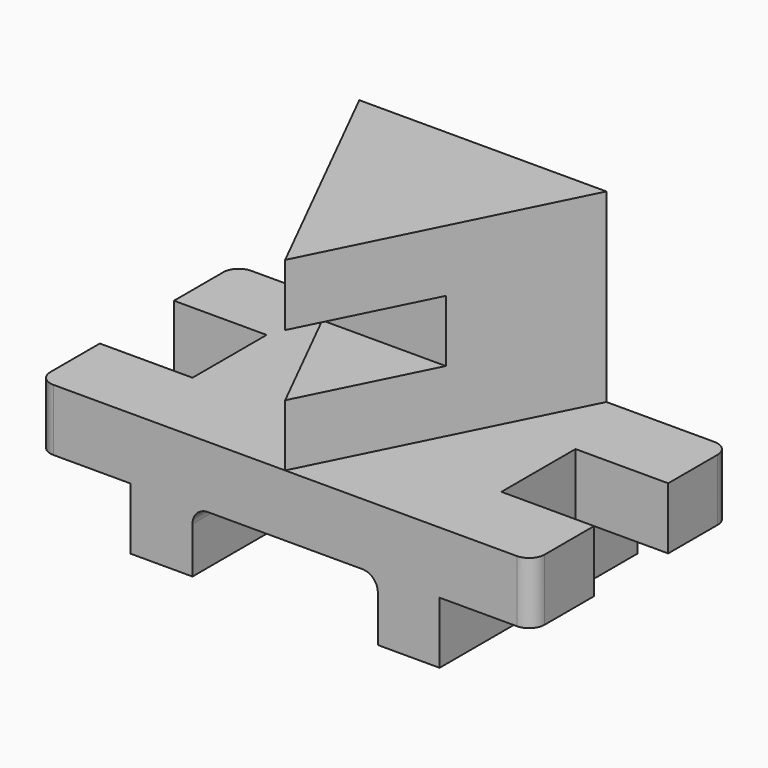
from build123d import *

# Parameters (mm, degrees)
F1_DEPTH = 25.4
F2_R     = 6.35
F4_DEPTH = 25.4
F5_R     = 6.35
F7_DEPTH = 76.2
F8_START = 25.4
F8_DEPTH = 25.4


with BuildPart() as f1:
    # F0 (on Top) → F1 (new body)
    with BuildSketch(Plane.XY):
        Polygon((-101.6, 19.05), (-63.5, 19.05), (-63.5, -19.05), (-101.6, -19.05), (-101.6, -50.8), (101.6, -50.8), (101.6, -19.05), (63.5, -19.05), (63.5, 19.05), (101.6, 19.05), (101.6, 50.8), (-101.6, 50.8), align=None)
    extrude(amount=-F1_DEPTH)

    # F2
    f2_edges = [f1.edges().sort_by_distance(p)[0] for p in [
        (-101.6, -50.8, -12.7),
        (101.6, -50.8, -12.7),
        (101.6, 50.8, -12.7),
        (-101.6, 50.8, -12.7),
    ]]
    fillet(f2_edges, radius=F2_R)

    # F3 (on face) → F4 (join)
    with BuildSketch(Plane(origin=(0, 0, -25.4), x_dir=(1, 0, 0), z_dir=(0, 0, -1))):
        Polygon((-38.1, -50.8), (-38.1, 50.8), (-63.5, 50.8), (-63.5, 19.05), (-63.5, -19.05), (-63.5, -50.8), align=None)
        Polygon((63.5, -19.05), (63.5, 19.05), (63.5, 50.8), (38.1, 50.8), (38.1, -50.8), (63.5, -50.8), align=None)
    extrude(amount=F4_DEPTH)

    # F5
    f5_edges = [f1.edges().sort_by_distance(p)[0] for p in [
        (-38.1, 0, -25.4),
        (38.1, 0, -25.4),
    ]]
    fillet(f5_edges, radius=F5_R)

    # F6 (on face) → F7 (join)
    with BuildSketch(Plane.XY):
        Polygon((-25.4, 0), (0, -50.8), (25.4, 0), (0, 0), align=None)
        Polygon((-50.8, 50.8), (-25.4, 0), (0, 0), (25.4, 0), (50.8, 50.8), align=None)
    extrude(amount=F7_DEPTH)

    # F6 (on face) → F8 (cut)
    with BuildSketch(Plane.XY.offset(F8_START)):
        Polygon((-25.4, 0), (0, -50.8), (25.4, 0), (0, 0), align=None)
    extrude(amount=F8_DEPTH, mode=Mode.SUBTRACT)


solid = f1.part
